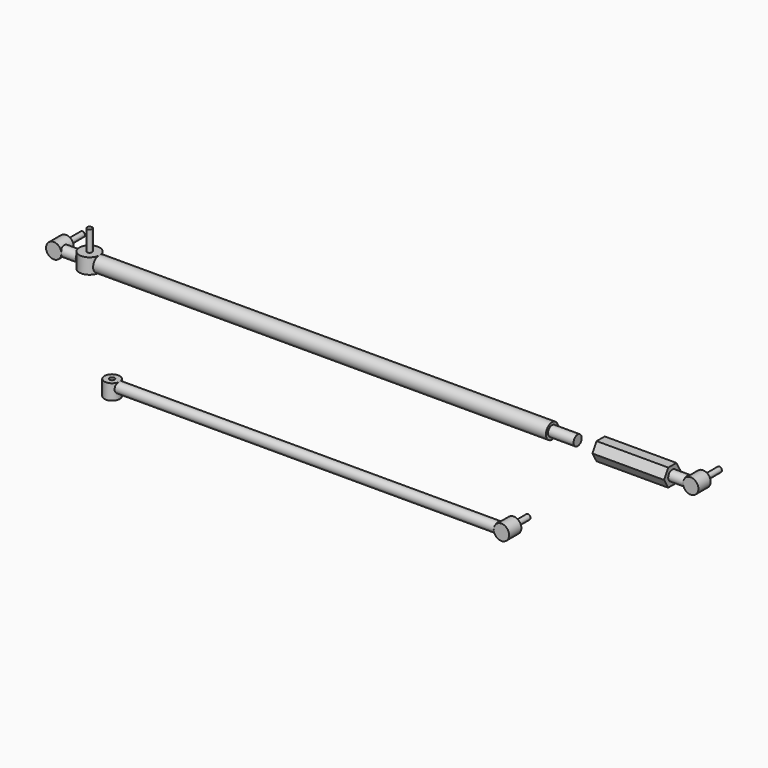
from build123d import *

# Parameters (mm, degrees)
F0_R      = 10
F1_DEPTH  = 140
F3_R      = 10
F4_DEPTH  = 70
F7_DEPTH  = 30
F9_DEPTH  = 60
F13_R     = 20
F14_DEPTH = 30
F15_R     = 5
F16_DEPTH = 55
F17_W     = 30
F17_H     = 10
F19_R     = 15
F20_DEPTH = 30
F21_R     = 5
F22_DEPTH = 60
F23_W     = 742
F23_H     = 10
F25_R     = 15
F26_DEPTH = 30
F27_R     = 5
F28_DEPTH = 55
F30_R     = 15
F30_R_2   = 5
F31_DEPTH = 30


with BuildPart() as f1:
    # F0 (on Right) → F1 (new body)
    with BuildSketch(Plane.YZ):
        Polygon((19.9997544387, -0.0991079843), (10.0857072515, 17.2707414212), (-9.9140471872, 17.3698494055), (-19.9997544387, 0.0991079843), (-10.0857072515, -17.2707414212), (9.9140471872, -17.3698494055), align=None)
        Circle(F0_R, mode=Mode.SUBTRACT)
    extrude(amount=F1_DEPTH)

    # F3 (on offset) → F4 (join)
    with BuildSketch(Plane.YZ.offset(100)):
        Circle(F3_R)
    extrude(amount=F4_DEPTH)

    # F6 (on offset) → F7 (join)
    with BuildSketch(Plane.XZ.offset(10)):
        with BuildLine():
            ThreePointArc((169, 0), (184, -15), (199, 0))
            ThreePointArc((199, 0), (184, 15), (169, 0))
        make_face()
    extrude(amount=-F7_DEPTH)


with BuildPart() as f9:
    # F8 (on Front) → F9 (new body)
    with BuildSketch(Plane.XZ):
        with BuildLine():
            ThreePointArc((179, 0), (184, -5), (189, 0))
            ThreePointArc((189, 0), (184, 5), (179, 0))
        make_face()
    extrude(amount=-F9_DEPTH)


with BuildPart() as f11:
    # F10 (on Front) → F11 (revolve)
    with BuildSketch(Plane.XZ):
        Polygon((-980, 0), (-45, 0), (-45, 10), (-95, 10), (-95, 15), (-980, 15), align=None)
    revolve(axis=Axis((-512.5, 0, 0), (-1, 0, 0)))

    # F13 (on offset) → F14 (join)
    with BuildSketch(Plane.XY.offset(15)):
        with Locations((-999, 0)):
            Circle(F13_R)
    extrude(amount=-F14_DEPTH)

    # F17 (on Top) → F18 (revolve)
    with BuildSketch(Plane.XY):
        with Locations((-1033, 5)):
            Rectangle(F17_W, F17_H)
    revolve(axis=Axis((-1033, 0, 0), (-1, 0, 0)))

    # F19 (on offset) → F20 (join)
    with BuildSketch(Plane.XZ.offset(10)):
        with Locations((-1061, 0)):
            Circle(F19_R)
    extrude(amount=-F20_DEPTH)


with BuildPart() as f16:
    # F15 (on Top) → F16 (new body)
    with BuildSketch(Plane.XY):
        with Locations((-999, 0)):
            Circle(F15_R)
    extrude(amount=F16_DEPTH)


with BuildPart() as f22:
    # F21 (on Front) → F22 (new body)
    with BuildSketch(Plane.XZ):
        with Locations((-1061, 0)):
            Circle(F21_R)
    extrude(amount=-F22_DEPTH)


with BuildPart() as f24:
    # F23 (on Front) → F24 (revolve)
    with BuildSketch(Plane.XZ):
        with Locations((-571, -195)):
            Rectangle(F23_W, F23_H)
    revolve(axis=Axis((-571, 0, -200), (-1, 0, 0)))

    # F25 (on offset) → F26 (join)
    with BuildSketch(Plane.XZ.offset(10)):
        with Locations((-186, -200)):
            Circle(F25_R)
    extrude(amount=-F26_DEPTH)

    # F30 (on offset) → F31 (join)
    with BuildSketch(Plane.XY.offset(-190)):
        with Locations((-955, 0)):
            Circle(F30_R)
        with Locations((-955, 0)):
            Circle(F30_R_2, mode=Mode.SUBTRACT)
    extrude(amount=-F31_DEPTH)


with BuildPart() as f28:
    # F27 (on Front) → F28 (new body)
    with BuildSketch(Plane.XZ):
        with Locations((-186, -200)):
            Circle(F27_R)
    extrude(amount=-F28_DEPTH)


solid = Compound([f1.part, f9.part, f11.part, f16.part, f22.part, f24.part, f28.part])
